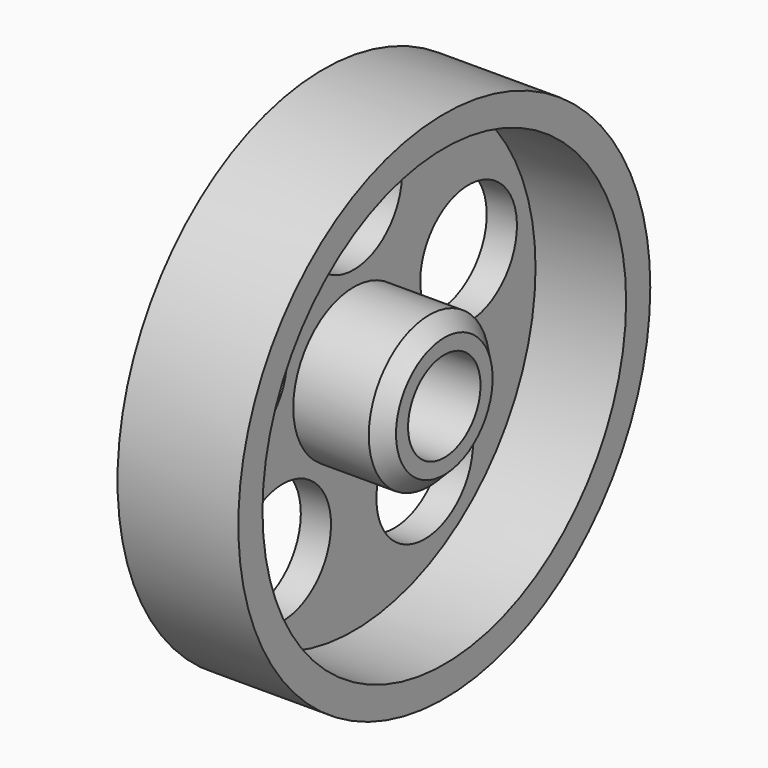
from build123d import *

# Parameters (mm, degrees)
F0_W            = 8
F0_H            = 17.05
F3_D            = 6
F4_T            = -2
F6_D            = 8
F6_COPIES_COUNT = 5
F7_SIZE         = 1


# Not quite as in the source:
# - a pattern or mirror of a feature is missing from the dataset's text; its kind, count and spacing are read off the source's solid


with BuildPart() as f1:
    # F0 (on Top) → F1 (revolve)
    with BuildSketch(Plane.XY):
        with Locations((4, 8.525)):
            Rectangle(F0_W, F0_H)
    revolve(axis=Axis((4, 0, 0), (1, 0, 0)))

    # F3 (through all)
    with Locations(Plane(origin=(0, 0, 0), x_dir=(0, 1, 0), z_dir=(-1, 0, 0))):
        with Locations((0, 0)):
            Hole(F3_D / 2)

    # F4
    f4_openings = [f1.faces().sort_by_distance(p)[0] for p in [
        (8, -16.567753, 0),
    ]]
    offset(amount=F4_T, openings=f4_openings)

    # F6 (through all)
    with Locations(Plane(origin=(0, 0, 0), x_dir=(0, 1, 0), z_dir=(-1, 0, 0))):
        with Locations((0, -10)):
            f6 = Hole(F6_D / 2)

    # F6_copies: F6 ×5 about axis
    f6_copies_axis = Axis((0, 0, 0), (1, 0, 0))
    for i in range(1, F6_COPIES_COUNT):
        add(f6.rotate(f6_copies_axis, i * 360 / F6_COPIES_COUNT), mode=Mode.SUBTRACT)

    # F7
    f7_edges = [f1.edges().sort_by_distance(p)[0] for p in [
        (8, -5, 0),
    ]]
    chamfer(f7_edges, length=F7_SIZE)


solid = f1.part
